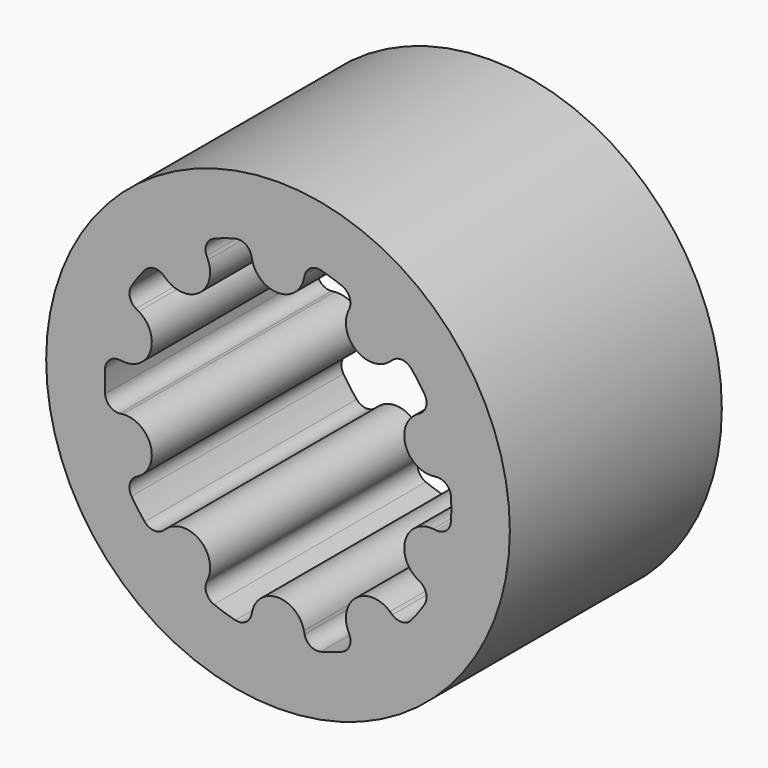
from build123d import *

# Parameters (mm, degrees)
F1_R            = 11.1125
F1_R_2          = 8.3058
F2_DEPTH        = 12.7
F4_DEPTH        = 12.7
F4_COPIES_COUNT = 10


# Not quite as in the source:
# - a pattern or mirror of a feature is missing from the dataset's text; its kind, count and spacing are read off the source's solid


with BuildPart() as f2:
    # F1 (on Front) → F2 (new body)
    with BuildSketch(Plane.XZ):
        Circle(F1_R)
        Circle(F1_R_2, mode=Mode.SUBTRACT)
    extrude(amount=F2_DEPTH)

    # F3 (on face) → F4 (join, through all)
    with BuildSketch(Plane(origin=(0, 0, 0), x_dir=(-1, 0, 0), z_dir=(0, 1, 0))):
        with BuildLine():
            ThreePointArc((-2.0497311639, 8.0489077393), (-1.5602325902, 7.9743573542), (-1.2730759239, 7.5709869752))
            Line((-1.2730759239, 7.5709869752), (-1.239895929, 7.4213216903))
            ThreePointArc((-1.239895929, 7.4213216903), (0, 6.4262), (1.239895929, 7.4213216903))
            Line((1.239895929, 7.4213216903), (1.2730759239, 7.5709869752))
            ThreePointArc((1.2730759239, 7.5709869752), (1.5602325902, 7.9743573542), (2.0497311639, 8.0489077393))
            ThreePointArc((2.0497311639, 8.0489077393), (0, 8.3058), (-2.0497311639, 8.0489077393))
        make_face()
    f4 = extrude(amount=-F4_DEPTH)

    # F4_copies: F4 ×10 about axis
    f4_copies_axis = Axis((0, 0, 0), (0, 1, 0))
    for i in range(1, F4_COPIES_COUNT):
        add(f4.rotate(f4_copies_axis, i * 360 / F4_COPIES_COUNT))


solid = f2.part
